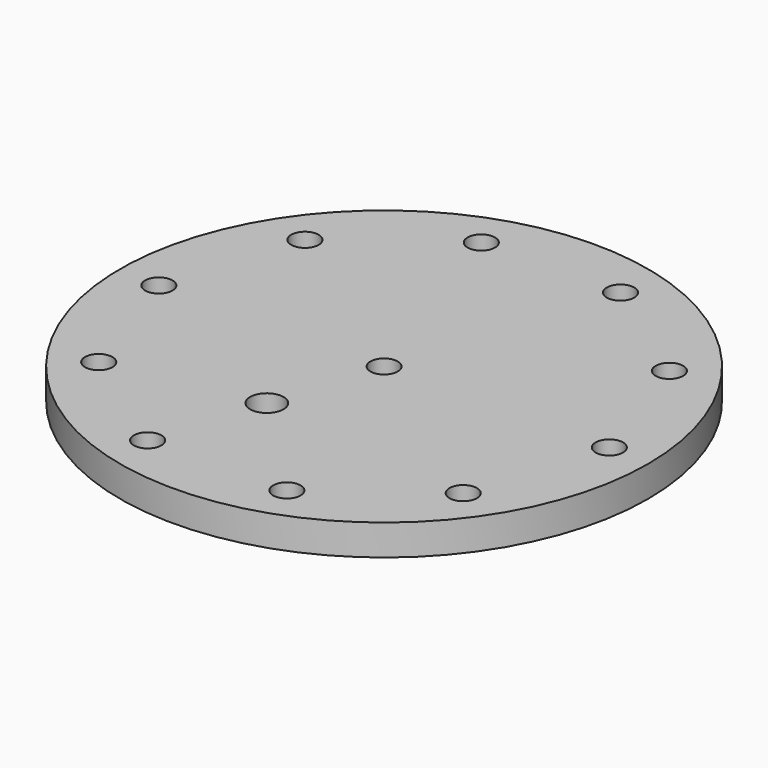
from build123d import *

# Parameters (mm, degrees)
F0_R            = 76.2
F1_DEPTH        = 8.89
F2_R            = 3.937
F3_DEPTH        = 25.4
F4_R            = 4.826
F5_DEPTH        = 25.4
F6_R            = 3.9624
F7_DEPTH        = 25.4
F7_COPIES_COUNT = 10


# Not quite as in the source:
# - a pattern or mirror of a feature is missing from the dataset's text; its kind, count and spacing are read off the source's solid


with BuildPart() as f1:
    # F0 (on Top) → F1 (new body)
    with BuildSketch(Plane.XY):
        Circle(F0_R)
    extrude(amount=F1_DEPTH)

    # F2 (on face) → F3 (cut)
    with BuildSketch(Plane.XY.offset(8.89)):
        Circle(F2_R)
    extrude(amount=-F3_DEPTH, mode=Mode.SUBTRACT)

    # F4 (on face) → F5 (cut)
    with BuildSketch(Plane.XY.offset(8.89)):
        with Locations((-9.46404, -30.48)):
            Circle(F4_R)
    extrude(amount=-F5_DEPTH, mode=Mode.SUBTRACT)

    # F6 (on face) → F7 (cut)
    with BuildSketch(Plane.XY.offset(8.89)):
        with Locations((-19.085301976, -61.4663509693)):
            Circle(F6_R)
    f7 = extrude(amount=-F7_DEPTH, mode=Mode.SUBTRACT)

    # F7_copies: F7 ×10 about axis
    f7_copies_axis = Axis((0, 0, 0), (0, 0, 1))
    for i in range(1, F7_COPIES_COUNT):
        add(f7.rotate(f7_copies_axis, i * 360 / F7_COPIES_COUNT), mode=Mode.SUBTRACT)


solid = f1.part
